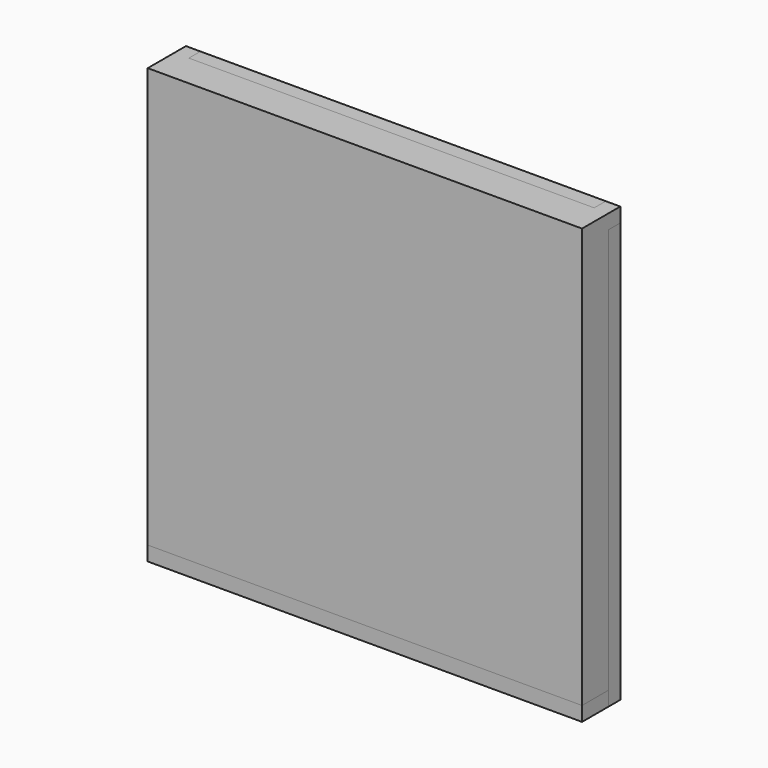
from build123d import *

# Parameters (mm, degrees)
F0_W      = 139.96
F0_H      = 139.96
F0_R      = 7.6
F1_DEPTH  = 3.5
F3_W      = 139.96
F3_H      = 139.96
F4_DEPTH  = 8
F7_DEPTH  = 11.5
F8_W      = 149.96
F8_H      = 5
F9_DEPTH  = 11.5
F10_W     = 5
F10_H     = 5
F11_DEPTH = 5
F13_DEPTH = 5


with BuildPart() as f1:
    # F0 (on Front) → F1 (new body)
    with BuildSketch(Plane.XZ):
        with Locations((-11.0969811678, -6.305641681)):
            Rectangle(F0_W, F0_H)
        with Locations((-61.0969811678, -56.305641681)):
            Circle(F0_R, mode=Mode.SUBTRACT)
        with Locations((-36.0969811678, -56.305641681)):
            Circle(F0_R, mode=Mode.SUBTRACT)
        with Locations((-61.0969811678, -31.305641681)):
            Circle(F0_R, mode=Mode.SUBTRACT)
        with Locations((-36.0969811678, -31.305641681)):
            Circle(F0_R, mode=Mode.SUBTRACT)
        with Locations((-11.0969811678, -56.305641681)):
            Circle(F0_R, mode=Mode.SUBTRACT)
        with Locations((13.9030188322, -56.305641681)):
            Circle(F0_R, mode=Mode.SUBTRACT)
        with Locations((38.9030188322, -56.305641681)):
            Circle(F0_R, mode=Mode.SUBTRACT)
        with Locations((-11.0969811678, -31.305641681)):
            Circle(F0_R, mode=Mode.SUBTRACT)
        with Locations((13.9030188322, -31.305641681)):
            Circle(F0_R, mode=Mode.SUBTRACT)
        with Locations((38.9030188322, -31.305641681)):
            Circle(F0_R, mode=Mode.SUBTRACT)
        with Locations((-61.0969811678, -6.305641681)):
            Circle(F0_R, mode=Mode.SUBTRACT)
        with Locations((-61.0969811678, 18.694358319)):
            Circle(F0_R, mode=Mode.SUBTRACT)
        with Locations((-36.0969811678, -6.305641681)):
            Circle(F0_R, mode=Mode.SUBTRACT)
        with Locations((-36.0969811678, 18.694358319)):
            Circle(F0_R, mode=Mode.SUBTRACT)
        with Locations((-61.0969811678, 43.694358319)):
            Circle(F0_R, mode=Mode.SUBTRACT)
        with Locations((-36.0969811678, 43.694358319)):
            Circle(F0_R, mode=Mode.SUBTRACT)
        with Locations((-11.0969811678, -6.305641681)):
            Circle(F0_R, mode=Mode.SUBTRACT)
        with Locations((13.9030188322, -6.305641681)):
            Circle(F0_R, mode=Mode.SUBTRACT)
        with Locations((-11.0969811678, 18.694358319)):
            Circle(F0_R, mode=Mode.SUBTRACT)
        with Locations((13.9030188322, 18.694358319)):
            Circle(F0_R, mode=Mode.SUBTRACT)
        with Locations((38.9030188322, -6.305641681)):
            Circle(F0_R, mode=Mode.SUBTRACT)
        with Locations((38.9030188322, 18.694358319)):
            Circle(F0_R, mode=Mode.SUBTRACT)
        with Locations((-11.0969811678, 43.694358319)):
            Circle(F0_R, mode=Mode.SUBTRACT)
        with Locations((13.9030188322, 43.694358319)):
            Circle(F0_R, mode=Mode.SUBTRACT)
        with Locations((38.9030188322, 43.694358319)):
            Circle(F0_R, mode=Mode.SUBTRACT)
    extrude(amount=F1_DEPTH)

    # F8 (on Front) → F9 (join)
    with BuildSketch(Plane.XZ):
        with Locations((-11.0969811678, -78.785641681)):
            Rectangle(F8_W, F8_H)
    extrude(amount=F9_DEPTH)


with BuildPart() as f4:
    # F3 (on offset) → F4 (new body)
    with BuildSketch(Plane.XZ.offset(3.5)):
        with Locations((-11.0969811678, -6.305641681)):
            Rectangle(F3_W, F3_H)
    extrude(amount=F4_DEPTH)

    # F6 (on offset) → F7 (join)
    with BuildSketch(Plane.XZ.offset(11.5)):
        Polygon((-81.0769811678, -76.285641681), (-81.0769811678, 63.674358319), (58.8830188322, 63.674358319), (58.8830188322, -76.285641681), (63.8830188322, -76.285641681), (63.8830188322, 68.674358319), (-86.0769811678, 68.674358319), (-86.0769811678, -76.285641681), align=None)
    extrude(amount=-F7_DEPTH)

    # F10 (on Front) → F11 (join)
    with BuildSketch(Plane.XZ):
        with Locations((-83.5769811678, 66.174358319)):
            Rectangle(F10_W, F10_H)
        with Locations((61.3830188322, 66.174358319)):
            Rectangle(F10_W, F10_H)
    extrude(amount=-F11_DEPTH)


with BuildPart() as f13:
    # F12 (on Front) → F13 (new body)
    with BuildSketch(Plane.XZ):
        Polygon((58.8830188322, 63.674358319), (58.8830188322, 68.674358319), (-81.0769811678, 68.674358319), (-81.0769811678, 63.674358319), (-86.0769811678, 63.674358319), (-86.0769811678, -81.285641681), (63.8830188322, -81.285641681), (63.8830188322, 63.674358319), align=None)
    extrude(amount=-F13_DEPTH)


solid = Compound([f1.part, f4.part, f13.part])
